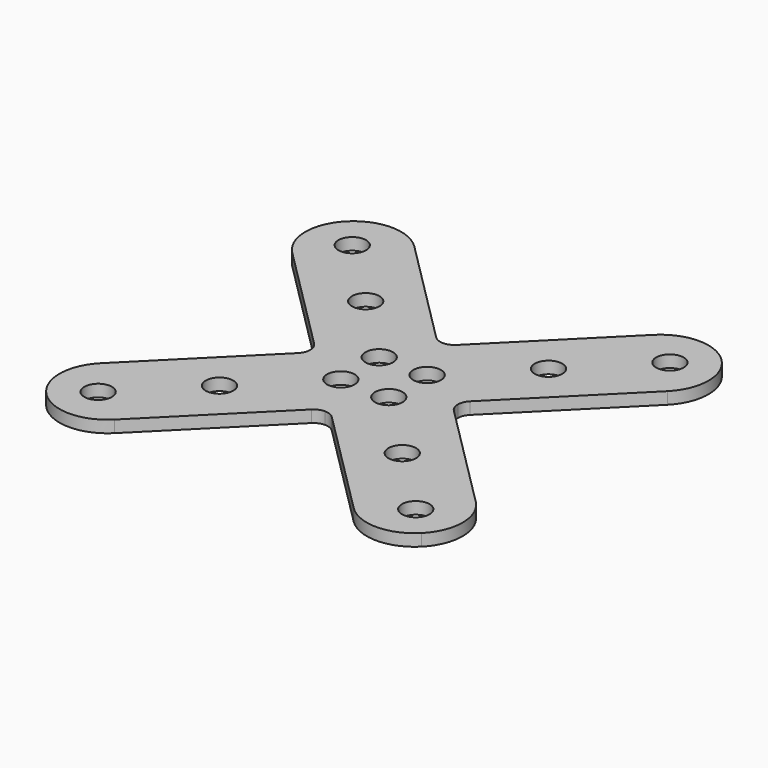
from build123d import *

# Parameters (mm, degrees)
F0_R     = 2.3
F1_DEPTH = 2
F4_R     = 7.99999
F5_R     = 2.4


# Not quite as in the source:
# - a fillet or chamfer is up to 0.001 mm smaller than in the source, because OpenCascade refuses the exact size


with BuildPart() as f1:
    # F0 (on Top) → F1 (new body)
    with BuildSketch(Plane.XY):
        Polygon((12.313708499, 1), (36.9456929209, 25.6319844219), (31.2888386714, 31.2888386714), (25.6319844219, 36.9456929209), (1, 12.313708499), (0, 11.313708499), (0, 0), (11.313708499, 0), align=None)
        with Locations((3.9999969952, 3.9999969952)):
            Circle(F0_R, mode=Mode.SUBTRACT)
        with Locations((15.2499951732, 15.2499951732)):
            Circle(F0_R, mode=Mode.SUBTRACT)
        with Locations((26.4999933512, 26.4999933512)):
            Circle(F0_R, mode=Mode.SUBTRACT)
        Polygon((0, 11.313708499), (1, 12.313708499), (0, 12.313708499), align=None)
        Polygon((12.313708499, 0), (12.313708499, 1), (11.313708499, 0), align=None)
    extrude(amount=F1_DEPTH)

    # F2: F1 across plane


with BuildPart() as f1_1:
    add(f1.part)
    add(f1.part.mirror(Plane.YZ))

    # F3: F1 across plane


with BuildPart() as f1_2:
    add(f1_1.part)
    add(f1_1.part.mirror(Plane.XZ))

    # F4 (radius 8 in the source; OpenCascade refuses exactly that, so slightly less here)
    f4_edges = [f1_2.edges().sort_by_distance(p)[0] for p in [
        (-25.631984, 36.945693, 1),
        (-36.945693, 25.631984, 1),
        (-36.945693, -25.631984, 1),
        (-25.631984, -36.945693, 1),
        (25.631984, -36.945693, 1),
        (36.945693, -25.631984, 1),
        (36.945693, 25.631984, 1),
        (25.631984, 36.945693, 1),
    ]]
    fillet(f4_edges, radius=F4_R)

    # F5
    f5_edges = [f1_2.edges().sort_by_distance(p)[0] for p in [
        (12.313708, 1, 1),
        (12.313708, -1, 1),
        (1, 12.313708, 1),
        (-1, 12.313708, 1),
        (-12.313708, 1, 1),
        (-12.313708, -1, 1),
        (-1, -12.313708, 1),
        (1, -12.313708, 1),
    ]]
    fillet(f5_edges, radius=F5_R)


solid = f1_2.part
